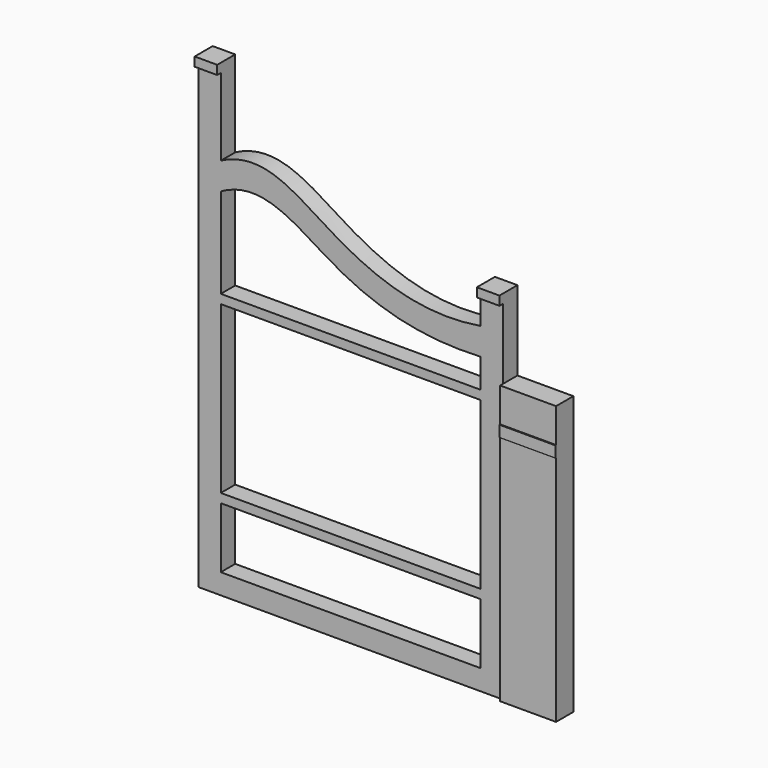
from build123d import *

# Parameters (mm, degrees)
F0_W     = 73.152
F0_H     = 5.744279672
F0_H_2   = 2.54
F1_DEPTH = 5.08
F0_W_2   = 6.35
F0_W_3   = 15.748
F0_H_3   = 3.1443536282
F2_DEPTH = 6.35
F0_H_4   = 65.5344708799
F0_H_5   = 9.6294713412
F3_DEPTH = 6.096


# Not quite as in the source:
# - a feature names something its author has since deleted; it is built from what else it names


with BuildPart() as f1:
    # F0 (on Front) → F1 (new body)
    with BuildSketch(Plane.XZ):
        Polygon((-44.2442491055, -63.1286278367), (-44.2442491055, -57.3843481647), (-44.2442491055, -40.2686278367), (-44.2442491055, -37.7286278367), (-44.2442491055, -32.8348538627), (-44.2442491055, -31.8823538627), (-44.2442491055, -30.9298538627), (-44.2442491055, -20.7698538627), (-44.2442491055, -19.8173538627), (-44.2442491055, -18.8648538627), (-44.2442491055, 9.1076644534), (-44.2442491055, 11.6476644534), (-44.2442491055, 15.1796680125), (-44.2442491055, 37.0476644534), (-44.2442491055, 44.6676644534), (-44.2442491055, 66.4113721633), (-50.5942491055, 66.4113721633), (-50.5942491055, -63.1286278367), align=None)
        with BuildLine():
            add(Edge.make_bspline(
                [(28.9077508945, 27.4595177274), (11.3712688144, 24.6047450509), (-13.4084815754, 35.2112312639), (-32.4729044871, 50.7994146886), (-44.2442491055, 44.6676644534)],
                knots=[0, 0, 0, 0, 0.5425588266, 1, 1, 1, 1], degree=3))
            Line((-44.2442491055, 44.6676644534), (-44.2442491055, 37.0476644534))
            add(Edge.make_bspline(
                [(28.9077508945, 19.8395177274), (11.5484302318, 18.9806314817), (-12.3449743232, 26.085082613), (-32.5652834278, 43.6948913941), (-44.2442491055, 37.0476644534)],
                knots=[0, 0, 0, 0, 0.5368571136, 1, 1, 1, 1], degree=3))
            Line((28.9077508945, 19.8395177274), (28.9077508945, 27.4595177274))
        make_face()
        Polygon((28.9077508945, -40.2686278367), (28.9077508945, -57.3843481647), (28.9077508945, -63.1286278367), (35.2577508945, -63.1286278367), (35.2577508945, 2.4058430432), (35.2577508945, 5.5501966713), (35.2577508945, 15.1796680125), (35.2577508945, 35.0404930887), (28.9077508945, 35.0404930887), (28.9077508945, 27.4595177274), (28.9077508945, 19.8395177274), (28.9077508945, 12.2195177274), (28.9077508945, 11.6476644534), (28.9077508945, 9.1076644534), (28.9077508945, -18.8648538627), (28.9077508945, -19.8173538627), (28.9077508945, -20.7698538627), (28.9077508945, -30.9298538627), (28.9077508945, -31.8823538627), (28.9077508945, -32.8348538627), (28.9077508945, -37.7286278367), align=None)
        with Locations((-7.6682491055, -60.2564880007)):
            Rectangle(F0_W, F0_H)
        with Locations((-7.6682491055, 10.3776644534)):
            Rectangle(F0_W, F0_H_2)
        with Locations((-7.6682491055, -38.9986278367)):
            Rectangle(F0_W, F0_H_2)
    extrude(amount=F1_DEPTH)

    # F0 (on Front) → F2 (join)
    with BuildSketch(Plane.XZ):
        with Locations((-47.4192491055, 67.6813721633)):
            Rectangle(F0_W_2, F0_H_2)
        with Locations((32.0827508945, 36.3104930887)):
            Rectangle(F0_W_2, F0_H_2)
        with Locations((43.1317508945, 3.9780198572)):
            Rectangle(F0_W_3, F0_H_3)
    extrude(amount=F2_DEPTH)

    # F0 (on Front) → F3 (join)
    with BuildSketch(Plane.XZ):
        with Locations((43.1317508945, -30.3613923968)):
            Rectangle(F0_W_3, F0_H_4)
        with Locations((43.1317508945, 10.3649323419)):
            Rectangle(F0_W_3, F0_H_5)
    extrude(amount=F3_DEPTH)


solid = f1.part
